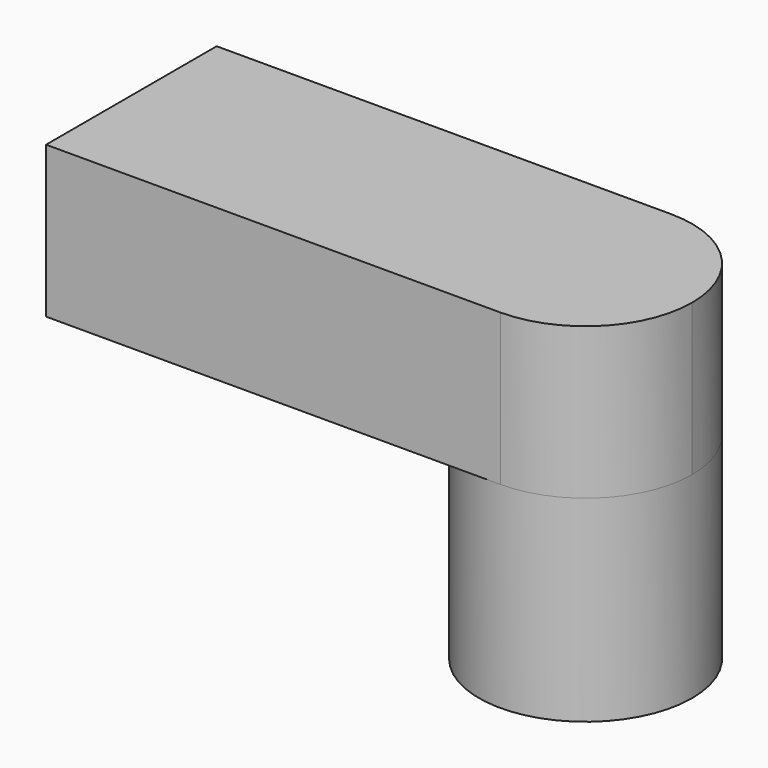
from build123d import *

# Parameters (mm, degrees)
F0_R     = 7.0414518843
F1_DEPTH = 3
F2_R     = 7.0414518843
F3_DEPTH = 10
F5_DEPTH = 10
F6_SIZE2 = 2.99999
F6_SIZE  = 0.49999


# Not quite as in the source:
# - a fillet or chamfer is up to 0.001 mm smaller than in the source, because OpenCascade refuses the exact size


with BuildPart() as f1:
    # F0 (on Top) → F1 (new body)
    with BuildSketch(Plane.XY):
        Circle(F0_R)
        Polygon((0, -4.0414518843), (-3.5, -2.0207259422), (-3.5, 2.0207259422), (0, 4.0414518843), (3.5, 2.0207259422), (3.5, -2.0207259422), align=None, mode=Mode.SUBTRACT)
    extrude(amount=F1_DEPTH)

    # F2 (on face) → F3 (join)
    with BuildSketch(Plane.XY.offset(3)):
        Circle(F2_R)
        Polygon((3.5, -2.0207259422), (0, -4.0414518843), (-3.5, -2.0207259422), (-3.5, 2.0207259422), (0, 4.0414518843), (3.5, 2.0207259422), align=None, mode=Mode.SUBTRACT)
        Polygon((-3.5, -2.0207259422), (0, -4.0414518843), (3.5, -2.0207259422), (3.5, 2.0207259422), (0, 4.0414518843), (-3.5, 2.0207259422), align=None)
    extrude(amount=F3_DEPTH)

    # F4 (on face) → F5 (join)
    with BuildSketch(Plane.XY.offset(13)):
        with BuildLine():
            ThreePointArc((7.0414518843, 0), (4.9790583768, 4.9790583768), (0, 7.0414518843))
            ThreePointArc((0, 7.0414518843), (-7.0414518843, 0), (0, -7.0414518843))
            ThreePointArc((0, -7.0414518843), (4.9790583768, -4.9790583768), (7.0414518843, 0))
        make_face()
        with BuildLine():
            ThreePointArc((0, -7.0414518843), (-7.0414518843, 0), (0, 7.0414518843))
            Line((0, 7.0414518843), (-30, 7.0414518843))
            Line((-30, 7.0414518843), (-30, -7.0414518843))
            Line((-30, -7.0414518843), (0, -7.0414518843))
        make_face()
    extrude(amount=F5_DEPTH)

    # F6 (size 0.5 and 3 in the source; OpenCascade refuses exactly that, so slightly less here)
    f6_edges = [f1.edges().sort_by_distance(p)[0] for p in [
        (-1.75, -3.031089, 0),
        (-3.5, 0, 0),
        (1.75, -3.031089, 0),
        (3.5, 0, 0),
        (1.75, 3.031089, 0),
        (-1.75, 3.031089, 0),
    ]]
    f6_side = f1.faces().sort_by_distance((-6.84229, 0, 0))[0]
    chamfer(f6_edges, length=F6_SIZE, length2=F6_SIZE2, reference=f6_side)


solid = f1.part
